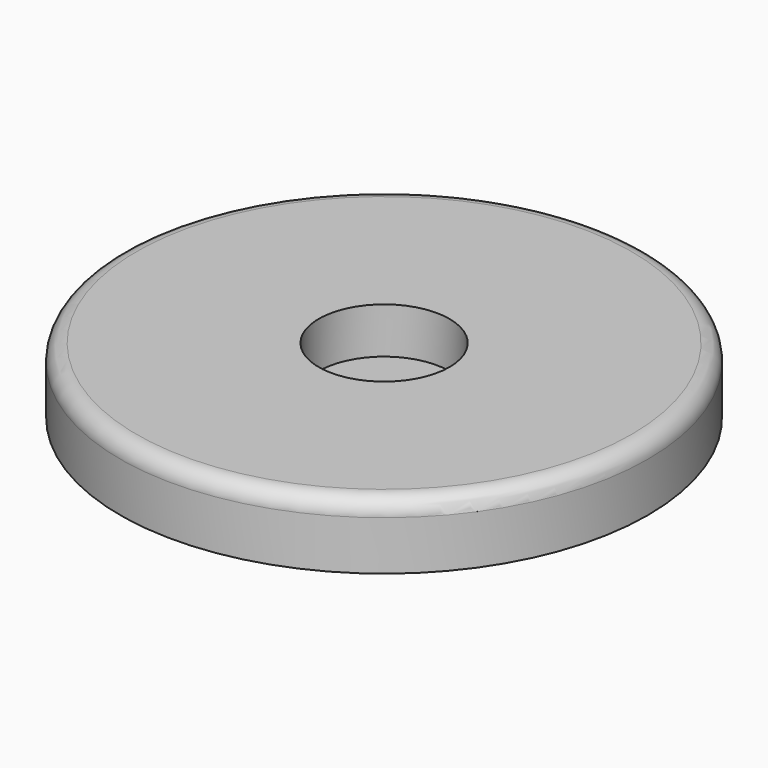
from build123d import *

# Parameters (mm, degrees)
F1_R     = 20.4097396771
F1_R_2   = 5.0527941738
F2_DEPTH = 5.08
F3_R     = 9.3754452045
F4_DEPTH = 1.524
F6_R     = 1.27


# Not quite as in the source:
# - a feature names something its author has since deleted; it is built from what else it names


with BuildPart() as f2:
    # F1 (on face) → F2 (new body)
    with BuildSketch(Plane.XY):
        Circle(F1_R)
        Circle(F1_R_2, mode=Mode.SUBTRACT)
    extrude(amount=F2_DEPTH)

    # F3 (on Top) → F4 (join)
    with BuildSketch(Plane.XY):
        Circle(F3_R)
    extrude(amount=F4_DEPTH)

    # F6
    f6_edges = [f2.edges().sort_by_distance(p)[0] for p in [
        (-20.40974, 0, 5.08),
    ]]
    fillet(f6_edges, radius=F6_R)


solid = f2.part
